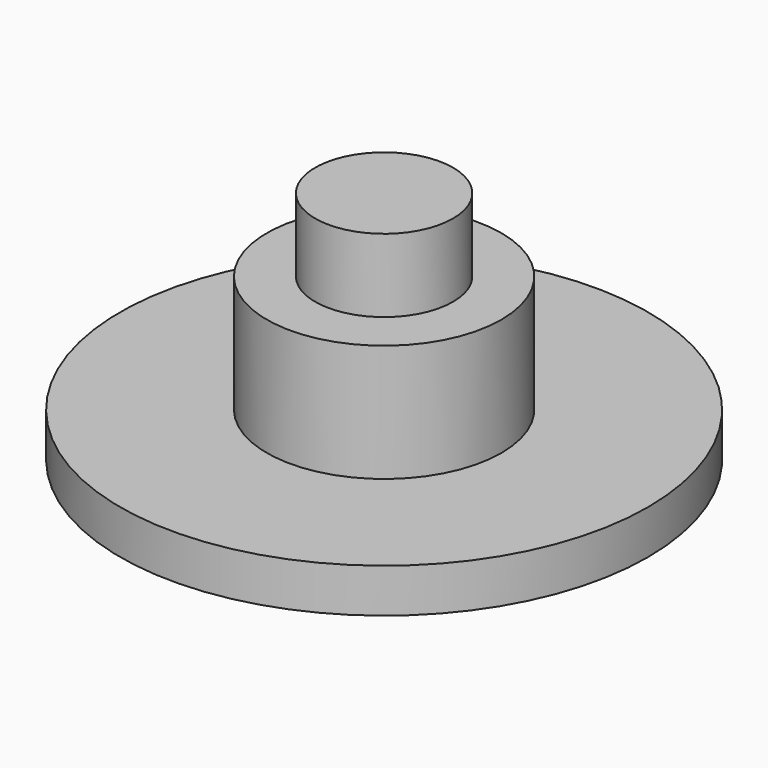
from build123d import *

# Parameters (mm, degrees)
F0_R     = 9
F0_R_2   = 4
F1_DEPTH = 1.5
F2_DEPTH = 4
F3_R     = 2.35
F4_DEPTH = 2.5


# Not quite as in the source:
# - a feature names something its author has since deleted; it is built from what else it names


with BuildPart() as f1:
    # F0 (on Top) → F1 (new body)
    with BuildSketch(Plane.XY):
        Circle(F0_R)
        Circle(F0_R_2, mode=Mode.SUBTRACT)
        Circle(F0_R_2)
    extrude(amount=-F1_DEPTH)

    # F0 (on Top) → F2 (join)
    with BuildSketch(Plane.XY):
        Circle(F0_R_2)
    extrude(amount=F2_DEPTH)

    # F3 (on face) → F4 (join)
    with BuildSketch(Plane.XY.offset(4)):
        Circle(F3_R)
    extrude(amount=F4_DEPTH)


solid = f1.part
